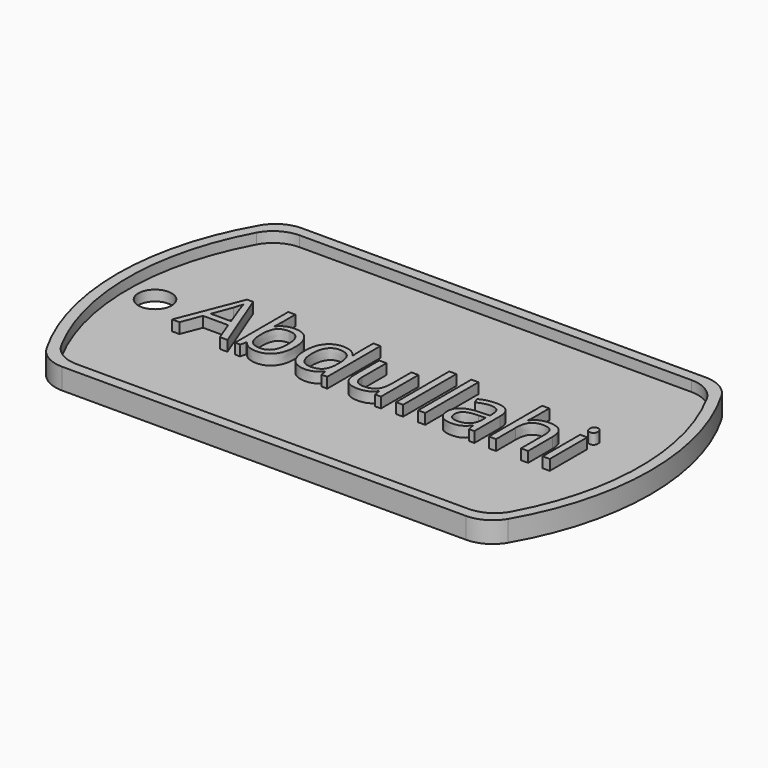
from build123d import *

# Parameters (mm, degrees)
F1_DEPTH     = 1
F3_DEPTH     = 1
F4_R         = 1.5875
F5_DEPTH     = 1
F7_TEXT_SIZE = 8.3404987688
F8_DEPTH     = 1


# Not quite as in the source:
# - Text() gives the source's letters only with a copy of the font that has no kerning and outlines rounded to 1/6400 em; it was checked with that copy


with BuildPart() as f1:
    # F0 (on Top) → F1 (new body)
    with BuildSketch(Plane.XY):
        with BuildLine():
            ThreePointArc((-19.2474145991, 14.2875), (-20.8349145991, 13.862130657), (-21.9970452561, 12.7))
            ThreePointArc((-21.9970452561, 12.7), (-25.4, 0), (-21.9970452561, -12.7))
            ThreePointArc((-21.9970452561, -12.7), (-20.8349145991, -13.862130657), (-19.2474145991, -14.2875))
            Line((-19.2474145991, -14.2875), (19.2474145991, -14.2875))
            ThreePointArc((19.2474145991, -14.2875), (20.8349145991, -13.862130657), (21.9970452561, -12.7))
            ThreePointArc((21.9970452561, -12.7), (25.4, 0), (21.9970452561, 12.7))
            ThreePointArc((21.9970452561, 12.7), (20.8349145991, 13.862130657), (19.2474145991, 14.2875))
            Line((19.2474145991, 14.2875), (-19.2474145991, 14.2875))
        make_face()
    extrude(amount=F1_DEPTH)

    # F2 (on face) → F3 (join)
    with BuildSketch(Plane.XY.offset(1)):
        with BuildLine():
            Line((19.2474145991, 14.2875), (-19.2474145991, 14.2875))
            ThreePointArc((-19.2474145991, 14.2875), (-20.8349145991, 13.862130657), (-21.9970452561, 12.7))
            ThreePointArc((-21.9970452561, 12.7), (-25.4, 0), (-21.9970452561, -12.7))
            ThreePointArc((-21.9970452561, -12.7), (-20.8349145991, -13.862130657), (-19.2474145991, -14.2875))
            Line((-19.2474145991, -14.2875), (19.2474145991, -14.2875))
            ThreePointArc((19.2474145991, -14.2875), (20.8349145991, -13.862130657), (21.9970452561, -12.7))
            ThreePointArc((21.9970452561, -12.7), (25.4, 0), (21.9970452561, 12.7))
            ThreePointArc((21.9970452561, 12.7), (20.8349145991, 13.862130657), (19.2474145991, 14.2875))
        make_face()
        with BuildLine():
            ThreePointArc((-21.4526124879, 11.6252061249), (-20.2856017842, 12.8404540819), (-18.6611352482, 13.2875))
            Line((-18.6611352482, 13.2875), (18.6611352482, 13.2875))
            ThreePointArc((18.6611352482, 13.2875), (20.2856017842, 12.8404540819), (21.4526124879, 11.6252061249))
            ThreePointArc((21.4526124879, 11.6252061249), (24.4, 0), (21.4526124879, -11.6252061249))
            ThreePointArc((21.4526124879, -11.6252061249), (20.2856017842, -12.8404540819), (18.6611352482, -13.2875))
            Line((18.6611352482, -13.2875), (-18.6611352482, -13.2875))
            ThreePointArc((-18.6611352482, -13.2875), (-20.2856017842, -12.8404540819), (-21.4526124879, -11.6252061249))
            ThreePointArc((-21.4526124879, -11.6252061249), (-24.4, 0), (-21.4526124879, 11.6252061249))
        make_face(mode=Mode.SUBTRACT)
    extrude(amount=F3_DEPTH)

    # F4 (on face) → F5 (cut)
    with BuildSketch(Plane.XY.offset(1)):
        with Locations((-21.821282804, 0)):
            Circle(F4_R)
    extrude(amount=-F5_DEPTH, mode=Mode.SUBTRACT)

    # F7 (on face) → F8 (join)
    with BuildSketch(Plane.XY.offset(1)):
        with Locations((-17.6119611133, -3.2256632112)):
            Text('Abdullahi', F7_TEXT_SIZE, font='Open Sans', text_align=(TextAlign.LEFT, TextAlign.BOTTOM))
    extrude(amount=F8_DEPTH)


solid = f1.part
